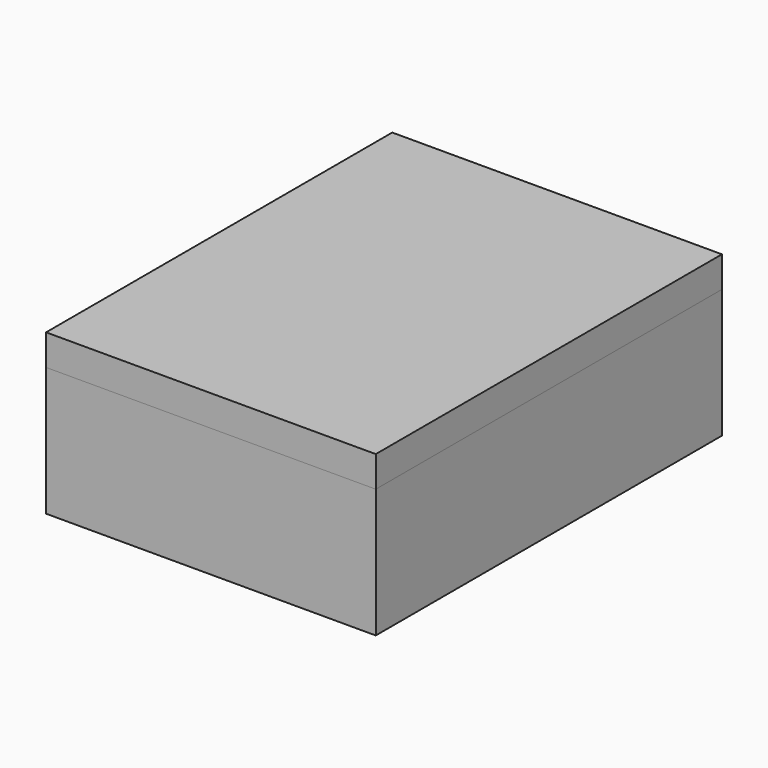
from build123d import *

# Parameters (mm, degrees)
F0_W     = 25.4
F0_H     = 9.921875
F1_DEPTH = 33.3375
F2_W     = 25.4
F2_H     = 2.38125
F3_DEPTH = 33.3375


# Not quite as in the source:
# - a feature names something its author has since deleted; it is built from what else it names


with BuildPart() as f1:
    # F0 (on Front) → F1 (new body)
    with BuildSketch(Plane.XZ):
        with Locations((12.7, 4.9609375)):
            Rectangle(F0_W, F0_H)
    extrude(amount=F1_DEPTH)


with BuildPart() as f3:
    # F2 (on Front) → F3 (new body)
    with BuildSketch(Plane.XZ):
        with Locations((12.7, 11.1125)):
            Rectangle(F2_W, F2_H)
    extrude(amount=F3_DEPTH)


solid = Compound([f1.part, f3.part])
